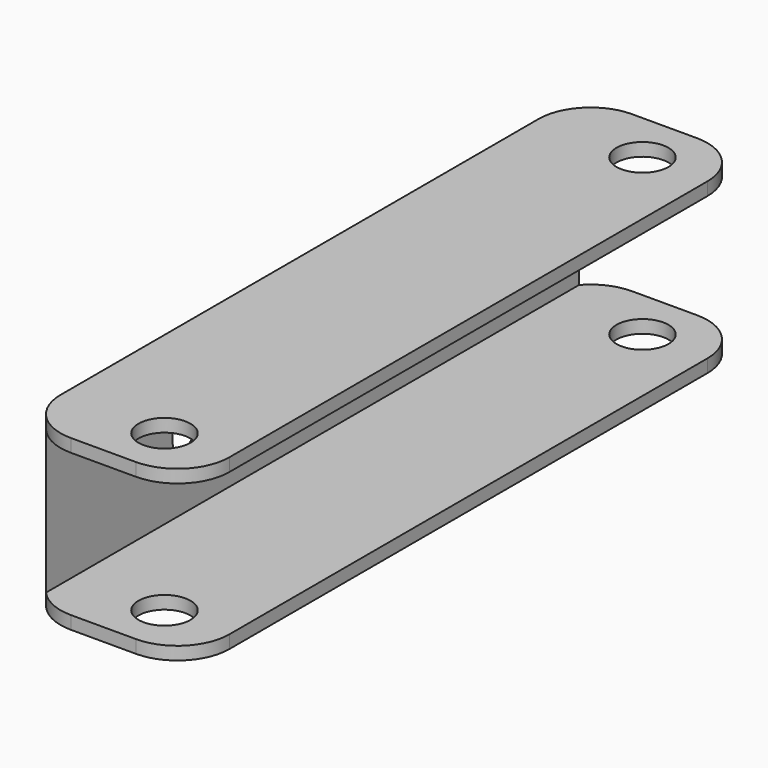
from build123d import *

# Parameters (mm, degrees)
F2_DEPTH    = 135
F1_R        = 5
F3_DEPTH    = 46
F4_T1_DEPTH = 52.5
F4_T3_DEPTH = 52.5
F4_T5_DEPTH = 82.5
F7_DEPTH    = 25


# Not quite as in the source:
# - a fillet or chamfer that OpenCascade refuses, or shapes differently, is made with other operations: its cross-section is extruded or revolved along the edge and cut away or added


with BuildPart() as f2:
    # F0 (on Front) → F2 (new body)
    with BuildSketch(Plane.XZ):
        Polygon((-74.9858543277, 32.5), (-74.9858543277, 0), (-42.4858543277, 0), (-42.4858543277, 2.5), (-72.4858543277, 2.5), (-72.4858543277, 30), (-42.4858543277, 30), (-42.4858543277, 32.5), align=None)
    extrude(amount=F2_DEPTH)

    # F1 (on Top) → F3 (cut)
    with BuildSketch(Plane.XY):
        with Locations((-54.9858543277, -260)):
            Circle(F1_R)
        with Locations((-54.9858543277, -125)):
            Circle(F1_R)
        with Locations((-54.9858543277, -10)):
            Circle(F1_R)
    extrude(amount=F3_DEPTH, mode=Mode.SUBTRACT)

    # F4: fillet of radius 10 on 6 edges, made by hand

    # F4_s2 → F4_t1 (cut)
    with BuildSketch(Plane.XY.offset(-25)):
        with BuildLine():
            ThreePointArc((-52.4858543277, 0), (-45.4147865158, -2.9289321881), (-42.4858543277, -10))
            Line((-42.4858543277, -10), (-42.4858543277, 0))
            Line((-42.4858543277, 0), (-52.4858543277, 0))
        make_face()
        with BuildLine():
            ThreePointArc((-52.4858543277, -135), (-45.4147865158, -132.0710678119), (-42.4858543277, -125))
            Line((-42.4858543277, -125), (-42.4858543277, -135))
            Line((-42.4858543277, -135), (-52.4858543277, -135))
        make_face()
    extrude(amount=F4_T1_DEPTH, mode=Mode.SUBTRACT)

    # F4_s4 → F4_t3 (cut)
    with BuildSketch(Plane.XY.offset(5)):
        with BuildLine():
            ThreePointArc((-42.4858543277, -10), (-45.4147865158, -2.9289321881), (-52.4858543277, 0))
            Line((-52.4858543277, 0), (-42.4858543277, 0))
            Line((-42.4858543277, 0), (-42.4858543277, -10))
        make_face()
        with BuildLine():
            ThreePointArc((-42.4858543277, -125), (-45.4147865158, -132.0710678119), (-52.4858543277, -135))
            Line((-52.4858543277, -135), (-42.4858543277, -135))
            Line((-42.4858543277, -135), (-42.4858543277, -125))
        make_face()
    extrude(amount=F4_T3_DEPTH, mode=Mode.SUBTRACT)

    # F4_s6 → F4_t5 (cut)
    with BuildSketch(Plane.XY.offset(-25)):
        with BuildLine():
            ThreePointArc((-64.9858543277, 0), (-72.0569221395, -2.9289321881), (-74.9858543277, -10))
            Line((-74.9858543277, -10), (-74.9858543277, 0))
            Line((-74.9858543277, 0), (-64.9858543277, 0))
        make_face()
        with BuildLine():
            ThreePointArc((-64.9858543277, -135), (-72.0569221395, -132.0710678119), (-74.9858543277, -125))
            Line((-74.9858543277, -125), (-74.9858543277, -135))
            Line((-74.9858543277, -135), (-64.9858543277, -135))
        make_face()
    extrude(amount=F4_T5_DEPTH, mode=Mode.SUBTRACT)

    # F6 (on offset) → F7 (cut)
    with BuildSketch(Plane(origin=(-74.9858543277, 0, 0), x_dir=(0, -1, 0), z_dir=(-1, 0, 0))):
        with BuildLine():
            Line((38.75, 16.25), (43.75, 16.25))
            ThreePointArc((43.75, 16.25), (35.2144660941, 19.7855339059), (38.75, 11.25))
            Line((38.75, 11.25), (38.75, 16.25))
        make_face()
        with BuildLine():
            ThreePointArc((38.75, 11.25), (42.2855339059, 12.7144660941), (43.75, 16.25))
            Line((43.75, 16.25), (38.75, 16.25))
            Line((38.75, 16.25), (38.75, 11.25))
        make_face()
        with BuildLine():
            ThreePointArc((101.25, 16.25), (96.25, 21.25), (91.25, 16.25))
            ThreePointArc((91.25, 16.25), (96.25, 11.25), (101.25, 16.25))
        make_face()
    extrude(amount=-F7_DEPTH, mode=Mode.SUBTRACT)


solid = f2.part
